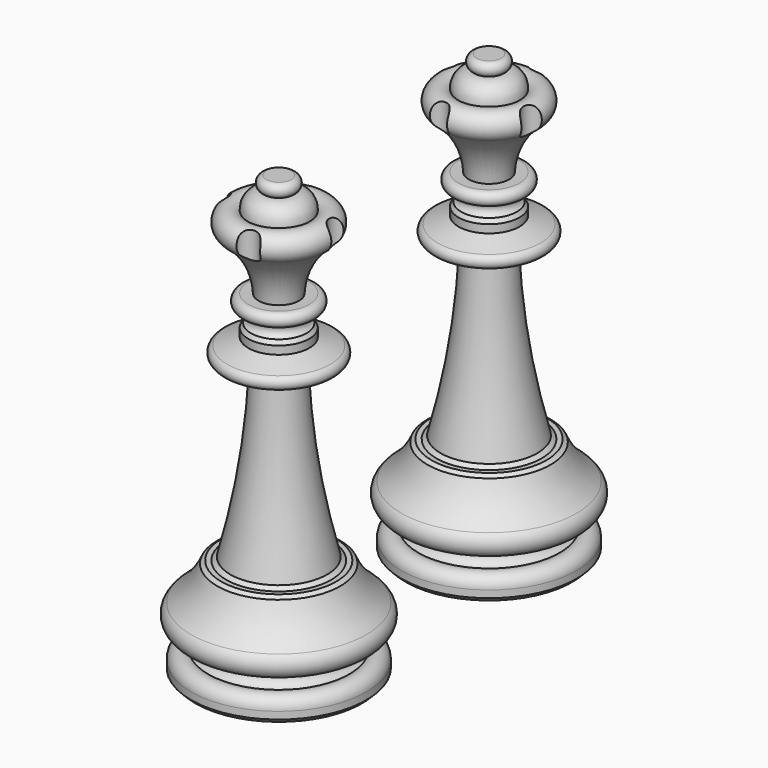
from build123d import *

# Parameters (mm, degrees)
F4_DEPTH = 25


# Not quite as in the source:
# - a fillet or chamfer that OpenCascade refuses, or shapes differently, is made with other operations: its cross-section is extruded or revolved along the edge and cut away or added


with BuildPart() as f1:
    # F0 (on Front) → F1 (revolve)
    with BuildSketch(Plane.XZ):
        with BuildLine():
            Line((-20, -47), (0, -47))
            Line((0, -47), (0, 53))
            Line((0, 53), (-2.8125754884, 53))
            ThreePointArc((-2.8125754884, 53), (-4.100798985, 51.466640085), (-2.8125754884, 49.93328017))
            ThreePointArc((-2.8125754884, 49.93328017), (-5.8482298192, 48.8987155336), (-6.9718565971, 45.8948872983))
            ThreePointArc((-6.9718565971, 45.8948872983), (-11.271804782, 45.594127893), (-10.99431701, 41.2926152349))
            ThreePointArc((-10.99431701, 41.2926152349), (-6.4142883123, 36.0047205702), (-4.609028806, 29.2460571689))
            Line((-4.609028806, 29.2460571689), (-6.9718565971, 29.2755700648))
            ThreePointArc((-6.9718565971, 29.2755700648), (-8.5252281914, 27.7414796874), (-6.9718565971, 26.20738931))
            ThreePointArc((-6.9718565971, 26.20738931), (-5.4199390172, 24.6951375157), (-6.9718565971, 23.1828857213))
            Line((-6.9718565971, 23.1828857213), (-6.9718565971, 20.5168376977))
            Line((-6.9718565971, 20.5168376977), (-11.7613635957, 18.7926143408))
            ThreePointArc((-11.7613635957, 18.7926143408), (-12.7497127989, 17.3863647506), (-11.7613635957, 15.9801151603))
            Line((-11.7613635957, 15.9801151603), (-5.3693195805, 13.6789781973))
            ThreePointArc((-5.3693195805, 13.6789781973), (-7.2397871389, -5.5344652894), (-11.2499995157, -24.4176127017))
            Line((-11.2499995157, -24.4176127017), (-13.8068180531, -24.4176127017))
            ThreePointArc((-13.8068180531, -24.4176127017), (-16.3242574251, -29.0614652929), (-20, -32.8551158309))
            ThreePointArc((-20, -32.8551158309), (-20.3551112115, -37.1022729576), (-16.1079540849, -37.4573841691))
            ThreePointArc((-16.1079540849, -37.4573841691), (-14.4493881554, -39.7585220635), (-16.1079540849, -42.0596599579))
            ThreePointArc((-16.1079540849, -42.0596599579), (-18.7103387647, -42.1000868461), (-20, -44.3607978523))
            Line((-20, -44.3607978523), (-20, -47))
        make_face()
    revolve(axis=Axis((0, 0, 61.6794213057), (0, 0, -1)))

    # F2: chamfer of 1 on 4 edges, made by hand

    # F2_s1 → F2_t2 (revolve)
    with BuildSketch(Plane.XZ):
        with BuildLine():
            Line((-11.0501054614, -23.6755661626), (-12.0162628047, -24.4176127017))
            Line((-12.0162628047, -24.4176127017), (-11.2499995157, -24.4176127017))
            ThreePointArc((-11.2499995157, -24.4176127017), (-11.1455065092, -24.031359988), (-11.0501054614, -23.6755661626))
        make_face()
    revolve(axis=Axis((0, 0, -24.4176127017), (0, 0, -1)))

    # F2_s3 → F2_t4 (revolve, cut)
    with BuildSketch(Plane.XZ):
        Polygon((-20, -46), (-19, -47), (-20, -47), align=None)
    revolve(axis=Axis((0, 0, -47), (0, 0, -1)), mode=Mode.SUBTRACT)

    # F2_s5 → F2_t6 (revolve, cut)
    with BuildSketch(Plane.XZ):
        with BuildLine():
            Line((-14.0508754504, -25.0333228188), (-13.1276629689, -24.4176127017))
            Line((-13.1276629689, -24.4176127017), (-13.8068180531, -24.4176127017))
            ThreePointArc((-13.8068180531, -24.4176127017), (-13.9322932992, -24.7418069322), (-14.0508754504, -25.0333228188))
        make_face()
    revolve(axis=Axis((0, 0, -24.4176127017), (0, 0, -1)), mode=Mode.SUBTRACT)

    # F2_s7 → F2_t8 (revolve, cut)
    with BuildSketch(Plane.XZ):
        with BuildLine():
            Line((-6.9718565971, 22.3733406577), (-6.354241553, 23.2973437668))
            ThreePointArc((-6.354241553, 23.2973437668), (-6.6428890598, 23.2103985337), (-6.9718565971, 23.1828857213))
            Line((-6.9718565971, 23.1828857213), (-6.9718565971, 22.3733406577))
        make_face()
    revolve(axis=Axis((0, 0, 23.1828857213), (0, 0, -1)), mode=Mode.SUBTRACT)

    # F3 (on face) → F4 (cut)
    with BuildSketch(Plane.XY.offset(53)):
        with BuildLine():
            ThreePointArc((-12.5, 0), (-9.7113426667, 1.9317061603), (-11.5484941564, 4.7835429046))
            Line((-11.5484941564, 4.7835429046), (-12.5, 0))
        make_face()
        with BuildLine():
            ThreePointArc((0, 12.5), (1.9317061603, 9.7113426667), (4.7835429046, 11.5484941564))
            Line((4.7835429046, 11.5484941564), (0, 12.5))
        make_face()
        with BuildLine():
            Line((11.5484941564, -4.7835429046), (12.5, 0))
            ThreePointArc((12.5, 0), (9.7113426667, -1.9317061603), (11.5484941564, -4.7835429046))
        make_face()
        with BuildLine():
            Line((-4.7835429046, -11.5484941564), (0, -12.5))
            ThreePointArc((0, -12.5), (-1.9317061603, -9.7113426667), (-4.7835429046, -11.5484941564))
        make_face()
    extrude(amount=-F4_DEPTH, mode=Mode.SUBTRACT)


with BuildPart() as f6_1:
    # F6: instance of F1
    add(f1.part.mirror(Plane.XZ.offset(30)))


solid = Compound([f1.part, f6_1.part])
